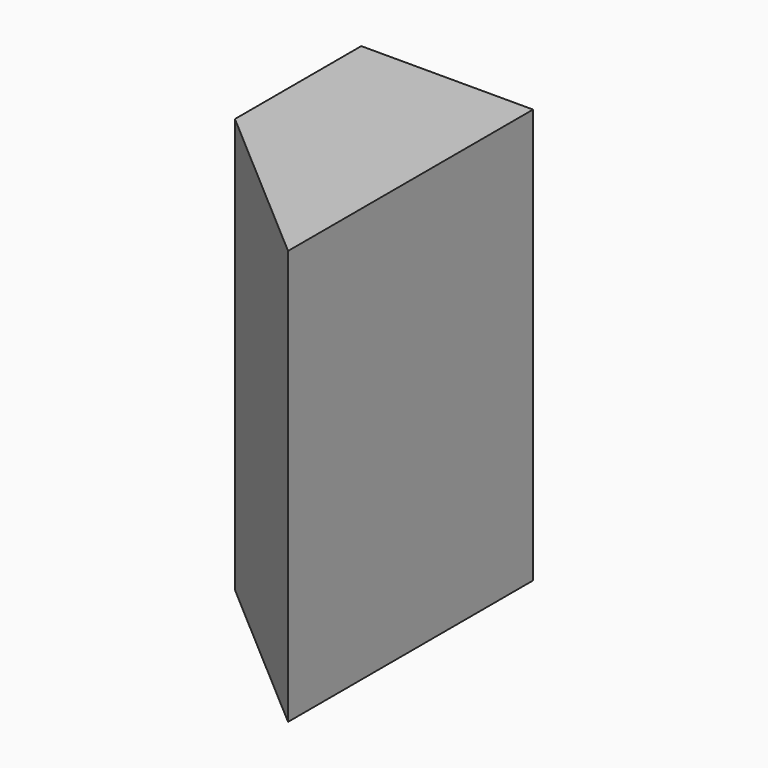
from build123d import *

# Parameters (mm, degrees)
F3_DEPTH = 228.6


# Not quite as in the source:
# - the program builds the solid bodies; features that only make, move or delete a surface that nothing else refers to are left out


with BuildPart() as f3:
    # F2 (on face) → F3 (new body)
    with BuildSketch(Plane.XY):
        Polygon((0, 87.0700776577), (0, 0), (94.7211682796, -81.7916764111), (94.7211682796, 87.0700776577), align=None)
    extrude(amount=F3_DEPTH)


solid = f3.part
